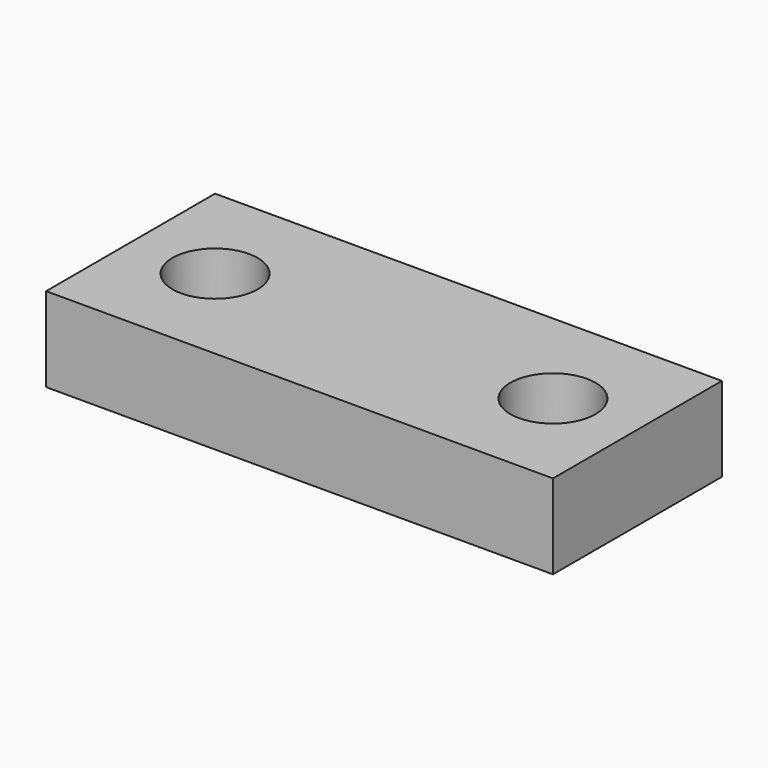
from build123d import *

# Parameters (mm, degrees)
F0_W     = 60
F0_H     = 10
F1_DEPTH = 12.5
F2_W     = 5.0413812651
F2_H     = 12


# Not quite as in the source:
# - a pattern or mirror of a feature is missing from the dataset's text; its kind, count and spacing are read off the source's solid


with BuildPart() as f1:
    # F0 (on Front) → F1 (new body, symmetric)
    with BuildSketch(Plane.XZ):
        with Locations((0, 5)):
            Rectangle(F0_W, F0_H)
    extrude(amount=F1_DEPTH, both=True)

    # F2 (on Front) → F3 (revolve, cut)
    with BuildSketch(Plane.XZ):
        with Locations((-22.5206906326, 6)):
            Rectangle(F2_W, F2_H)
    f3 = revolve(axis=Axis((-20, 0, 6), (0, 0, 1)), mode=Mode.SUBTRACT)

    # F3_copies: F3 across plane
    add(f3.mirror(Plane(origin=(0, 0, 0), x_dir=(0, 0, 1), z_dir=(1, 0, 0))), mode=Mode.SUBTRACT)


solid = f1.part
